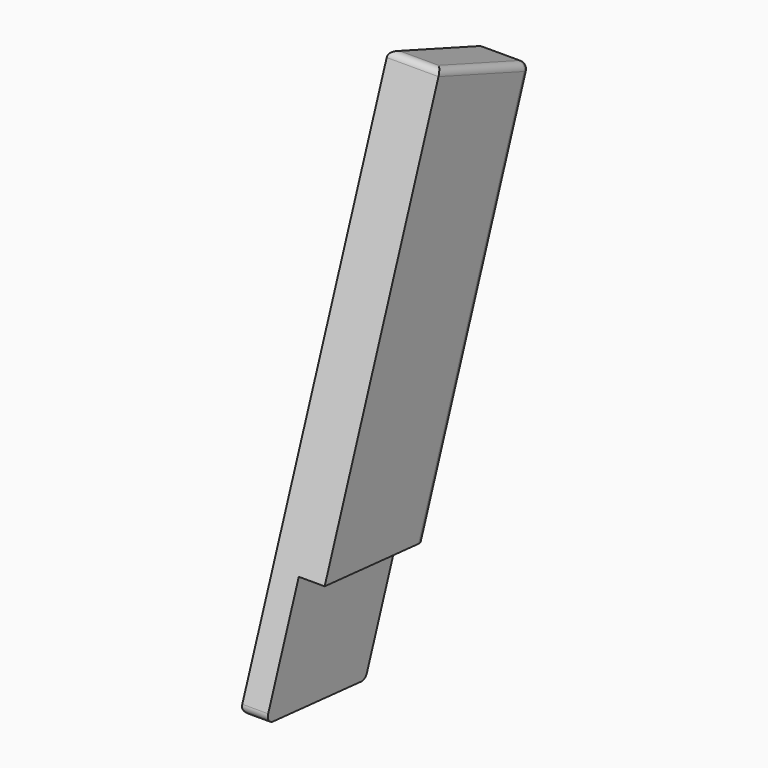
from build123d import *

# Parameters (mm, degrees)
F1_DEPTH = 38.1
F3_DEPTH = 19.05
F4_R     = 5.08


# Not quite as in the source:
# - a feature names something its author has since deleted; it is built from what else it names


with BuildPart() as f1:
    # F0 (on Right) → F1 (new body)
    with BuildSketch(Plane.YZ):
        Polygon((-91.6858274725, 8.0214705098), (0, 0), (128.6780048528, 353.5399127136), (45.1393308649, 383.9455034552), align=None)
    extrude(amount=F1_DEPTH)

    # F2 (on face) → F3 (cut)
    with BuildSketch(Plane.YZ.offset(38.1)):
        Polygon((-92.758420577, 5.074545175), (34.3168153471, -6.0430973832), (0, 0), (30.4055907417, 83.5386739879), (-61.2802367308, 91.5601444977), align=None)
    extrude(amount=-F3_DEPTH, mode=Mode.SUBTRACT)

    # F4
    f4_edges = [f1.edges().sort_by_distance(p)[0] for p in [
        (0, 86.908668, 368.742708),
        (0, 64.339002, 176.769956),
        (38.1, 79.541798, 218.539293),
        (9.525, 0, 0),
        (0, -45.842914, 4.010735),
        (9.525, -91.685827, 8.021471),
        (38.1, 86.908668, 368.742708),
        (19.05, 128.678005, 353.539913),
        (19.05, 45.139331, 383.945503),
    ]]
    fillet(f4_edges, radius=F4_R)


solid = f1.part
